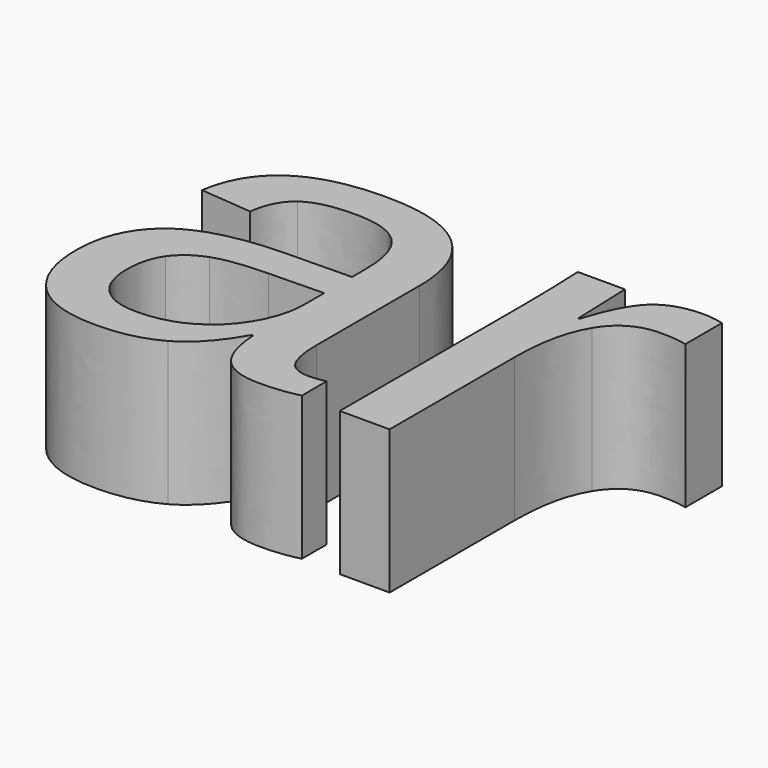
from build123d import *

# Parameters (mm, degrees)
F1_DEPTH = 25.4


with BuildPart() as f1:
    # F0 (on Top) → F1 (new body)
    with BuildSketch(Plane.XY):
        with BuildLine():
            Line((31.2962190364, 19.3968032254), (31.2962190364, -21.2388634682))
            Line((31.2962190364, -21.2388634682), (40.1000913116, -21.2388634682))
            Line((40.1000913116, -21.2388634682), (40.1000913116, 6.3789778505))
            add(Edge.make_bspline(
                [(42.9903305194, 19.905923953), (40.1000913116, 15.1828501257), (40.1000913116, 6.3789778505)],
                knots=[0, 0, 0, 1, 1, 1], degree=2))
            add(Edge.make_bspline(
                [(51.3634083327, 24.6289977804), (45.8805697272, 24.6289977804), (42.9903305194, 19.905923953)],
                knots=[0, 0, 0, 1, 1, 1], degree=2))
            add(Edge.make_bspline(
                [(56.0629842803, 24.1433749325), (54.3084759265, 24.6289977804), (51.3634083327, 24.6289977804)],
                knots=[0, 0, 0, 1, 1, 1], degree=2))
            Line((56.0629842803, 24.1433749325), (56.0629842803, 32.2266455623))
            add(Edge.make_bspline(
                [(52.4913065601, 32.7122684103), (54.2458149139, 32.7122684103), (56.0629842803, 32.2266455623)],
                knots=[0, 0, 0, 1, 1, 1], degree=2))
            add(Edge.make_bspline(
                [(44.7526714997, 30.2136605314), (47.4940908025, 32.7122684103), (52.4913065601, 32.7122684103)],
                knots=[0, 0, 0, 1, 1, 1], degree=2))
            add(Edge.make_bspline(
                [(39.9121082737, 20.9163327818), (42.011252197, 27.7150526526), (44.7526714997, 30.2136605314)],
                knots=[0, 0, 0, 1, 1, 1], degree=2))
            Line((39.9121082737, 20.9163327818), (39.7084599826, 20.9163327818))
            add(Edge.make_bspline(
                [(39.3168286537, 31.7253574613), (39.7084599826, 22.717836895), (39.7084599826, 20.9163327818)],
                knots=[0, 0, 0, 1, 1, 1], degree=2))
            Line((39.3168286537, 31.7253574613), (30.9985792264, 31.7253574613))
            add(Edge.make_bspline(
                [(31.2962190364, 19.3968032254), (31.2962190364, 24.9736333499), (30.9985792264, 31.7253574613)],
                knots=[0, 0, 0, 1, 1, 1], degree=2))
        make_face()
        with BuildLine():
            add(Edge.make_bspline(
                [(-11.1409517704, -22.2257744172), (-19.1302308813, -22.2257744172), (-23.1405356899, -18.0118213175)],
                knots=[0, 0, 0, 1, 1, 1], degree=2))
            add(Edge.make_bspline(
                [(-0.2536008251, -19.7036686586), (-4.7338632285, -22.2257744172), (-11.1409517704, -22.2257744172)],
                knots=[0, 0, 0, 1, 1, 1], degree=2))
            add(Edge.make_bspline(
                [(7.6103562606, -11.1034446745), (4.2266615783, -17.1815629001), (-0.2536008251, -19.7036686586)],
                knots=[0, 0, 0, 1, 1, 1], degree=2))
            Line((7.6103562606, -11.1034446745), (7.8923308174, -11.1034446745))
            add(Edge.make_bspline(
                [(10.4222692025, -19.1553847981), (8.1899706274, -16.58628328), (7.8923308174, -11.1034446745)],
                knots=[0, 0, 0, 1, 1, 1], degree=2))
            add(Edge.make_bspline(
                [(17.5421267631, -21.7244863161), (12.6545677776, -21.7244863161), (10.4222692025, -19.1553847981)],
                knots=[0, 0, 0, 1, 1, 1], degree=2))
            add(Edge.make_bspline(
                [(24.340846634, -20.9412236582), (21.0198129644, -21.7244863161), (17.5421267631, -21.7244863161)],
                knots=[0, 0, 0, 1, 1, 1], degree=2))
            Line((24.340846634, -20.9412236582), (24.340846634, -15.4583850526))
            add(Edge.make_bspline(
                [(21.4584400528, -15.8030206221), (22.7273255587, -15.8030206221), (24.340846634, -15.4583850526)],
                knots=[0, 0, 0, 1, 1, 1], degree=2))
            add(Edge.make_bspline(
                [(17.5421267631, -13.8213660975), (18.5760334716, -15.8030206221), (21.4584400528, -15.8030206221)],
                knots=[0, 0, 0, 1, 1, 1], degree=2))
            add(Edge.make_bspline(
                [(16.5082200547, -7.9233982833), (16.5082200547, -11.839711573), (17.5421267631, -13.8213660975)],
                knots=[0, 0, 0, 1, 1, 1], degree=2))
            Line((16.5082200547, -7.9233982833), (16.5082200547, 14.8852103157))
            add(Edge.make_bspline(
                [(11.4718411642, 28.1301818613), (16.5082200547, 23.5480953124), (16.5082200547, 14.8852103157)],
                knots=[0, 0, 0, 1, 1, 1], degree=2))
            add(Edge.make_bspline(
                [(-3.5589692416, 32.7122684103), (6.4354622737, 32.7122684103), (11.4718411642, 28.1301818613)],
                knots=[0, 0, 0, 1, 1, 1], degree=2))
            add(Edge.make_bspline(
                [(-24.8010525247, 18.4098922764), (-22.5452560699, 32.7122684103), (-3.5589692416, 32.7122684103)],
                knots=[0, 0, 0, 1, 1, 1], degree=2))
            Line((-24.8010525247, 18.4098922764), (-15.6055489206, 17.579633859))
            add(Edge.make_bspline(
                [(-12.3628415167, 23.9945550275), (-15.05726506, 21.9815699966), (-15.6055489206, 17.579633859)],
                knots=[0, 0, 0, 1, 1, 1], degree=2))
            add(Edge.make_bspline(
                [(-3.7469522795, 26.0075400583), (-9.6684179734, 26.0075400583), (-12.3628415167, 23.9945550275)],
                knots=[0, 0, 0, 1, 1, 1], degree=2))
            add(Edge.make_bspline(
                [(4.8689369578, 23.2112923695), (2.127517655, 26.0075400583), (-3.7469522795, 26.0075400583)],
                knots=[0, 0, 0, 1, 1, 1], degree=2))
            add(Edge.make_bspline(
                [(7.6103562606, 13.9609603793), (7.6103562606, 20.4150446807), (4.8689369578, 23.2112923695)],
                knots=[0, 0, 0, 1, 1, 1], degree=2))
            Line((7.6103562606, 13.9609603793), (7.6103562606, 11.0785537981))
            Line((7.6103562606, 11.0785537981), (-4.29523614, 10.8749055071))
            add(Edge.make_bspline(
                [(-21.7384955322, 6.1753295595), (-16.3261505659, 10.5772656971), (-4.29523614, 10.8749055071)],
                knots=[0, 0, 0, 1, 1, 1], degree=2))
            add(Edge.make_bspline(
                [(-27.1508404985, -6.4508644864), (-27.1508404985, 1.7733934219), (-21.7384955322, 6.1753295595)],
                knots=[0, 0, 0, 1, 1, 1], degree=2))
            add(Edge.make_bspline(
                [(-23.1405356899, -18.0118213175), (-27.1508404985, -13.7978682178), (-27.1508404985, -6.4508644864)],
                knots=[0, 0, 0, 1, 1, 1], degree=2))
        make_face()
        with BuildLine():
            add(Edge.make_bspline(
                [(-9.135799366, -15.6150375842), (-4.29523614, -15.6150375842), (-0.5199101288, -13.4062368888)],
                knots=[0, 0, 0, 1, 1, 1], degree=2))
            add(Edge.make_bspline(
                [(-15.7700340787, -13.2652496104), (-13.4437439847, -15.6150375842), (-9.135799366, -15.6150375842)],
                knots=[0, 0, 0, 1, 1, 1], degree=2))
            add(Edge.make_bspline(
                [(-18.0963241728, -6.607517018), (-18.0963241728, -10.9154616366), (-15.7700340787, -13.2652496104)],
                knots=[0, 0, 0, 1, 1, 1], degree=2))
            add(Edge.make_bspline(
                [(-16.3809789519, -0.1847632229), (-18.0963241728, -2.6285427157), (-18.0963241728, -6.607517018)],
                knots=[0, 0, 0, 1, 1, 1], degree=2))
            add(Edge.make_bspline(
                [(-11.4620894601, 3.4339102567), (-14.6656337311, 2.2590162698), (-16.3809789519, -0.1847632229)],
                knots=[0, 0, 0, 1, 1, 1], degree=2))
            add(Edge.make_bspline(
                [(-2.0394396852, 4.7027957626), (-8.2585451892, 4.6088042436), (-11.4620894601, 3.4339102567)],
                knots=[0, 0, 0, 1, 1, 1], degree=2))
            Line((-2.0394396852, 4.7027957626), (7.6103562606, 4.9064440536))
            Line((7.6103562606, 4.9064440536), (7.6103562606, 0.5515036755))
            add(Edge.make_bspline(
                [(5.4328860715, -7.3594491696), (7.6103562606, -3.5214621457), (7.6103562606, 0.5515036755)],
                knots=[0, 0, 0, 1, 1, 1], degree=2))
            add(Edge.make_bspline(
                [(-0.5199101288, -13.4062368888), (3.2554158824, -11.1974361935), (5.4328860715, -7.3594491696)],
                knots=[0, 0, 0, 1, 1, 1], degree=2))
        make_face(mode=Mode.SUBTRACT)
    extrude(amount=F1_DEPTH)


solid = f1.part
